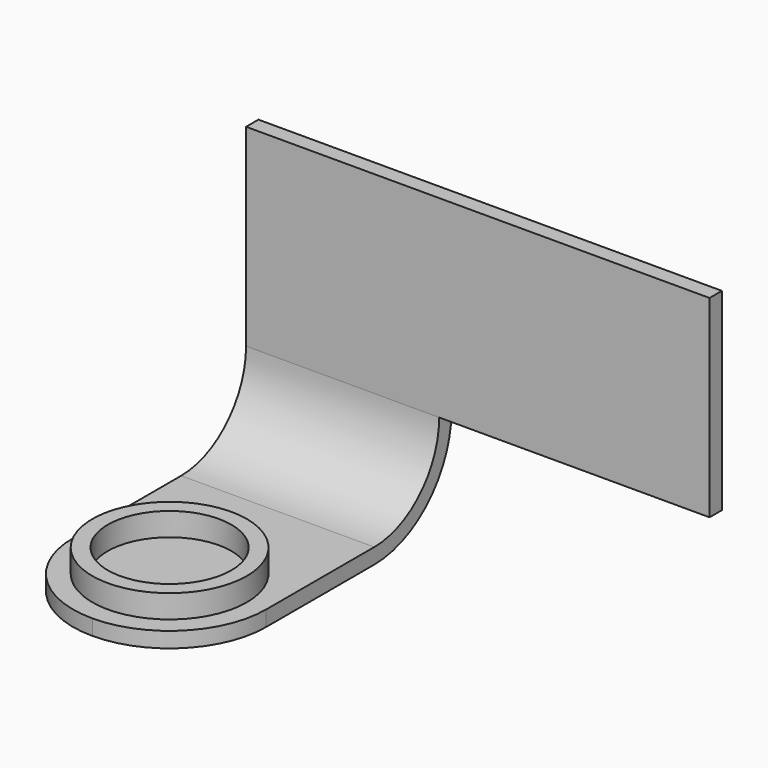
from build123d import *

# Parameters (mm, degrees)
F0_W     = 60
F0_H     = 25
F1_DEPTH = 2
F3_DEPTH = 12.5
F4_R     = 12.49999
F5_R     = 10
F5_R_2   = 8
F6_DEPTH = 3


# Not quite as in the source:
# - a fillet or chamfer is up to 0.001 mm smaller than in the source, because OpenCascade refuses the exact size


with BuildPart() as f1:
    # F0 (on Front) → F1 (new body)
    with BuildSketch(Plane.XZ):
        with Locations((17.5, 12.5)):
            Rectangle(F0_W, F0_H)
    extrude(amount=F1_DEPTH)

    # F2 (on Right) → F3 (join, symmetric)
    with BuildSketch(Plane.YZ):
        with BuildLine():
            Line((-42.5, -12.5), (-12.5, -12.5))
            ThreePointArc((-12.5, -12.5), (-3.6611652352, -8.8388347648), (0, 0))
            Line((0, 0), (-2, 0))
            ThreePointArc((-2, 0), (-5.0753787975, -7.4246212025), (-12.5, -10.5))
            Line((-12.5, -10.5), (-42.5, -10.5))
            Line((-42.5, -10.5), (-42.5, -12.5))
        make_face()
    extrude(amount=F3_DEPTH, both=True)

    # F4 (radius 12.5 in the source; OpenCascade refuses exactly that, so slightly less here)
    f4_edges = [f1.edges().sort_by_distance(p)[0] for p in [
        (-12.5, -42.5, -11.5),
        (12.5, -42.5, -11.5),
    ]]
    fillet(f4_edges, radius=F4_R)

    # F5 (on face) → F6 (join)
    with BuildSketch(Plane.XY.offset(-10.5)):
        with Locations((0, -30)):
            Circle(F5_R)
        with Locations((0, -30)):
            Circle(F5_R_2, mode=Mode.SUBTRACT)
    extrude(amount=F6_DEPTH)


solid = f1.part
